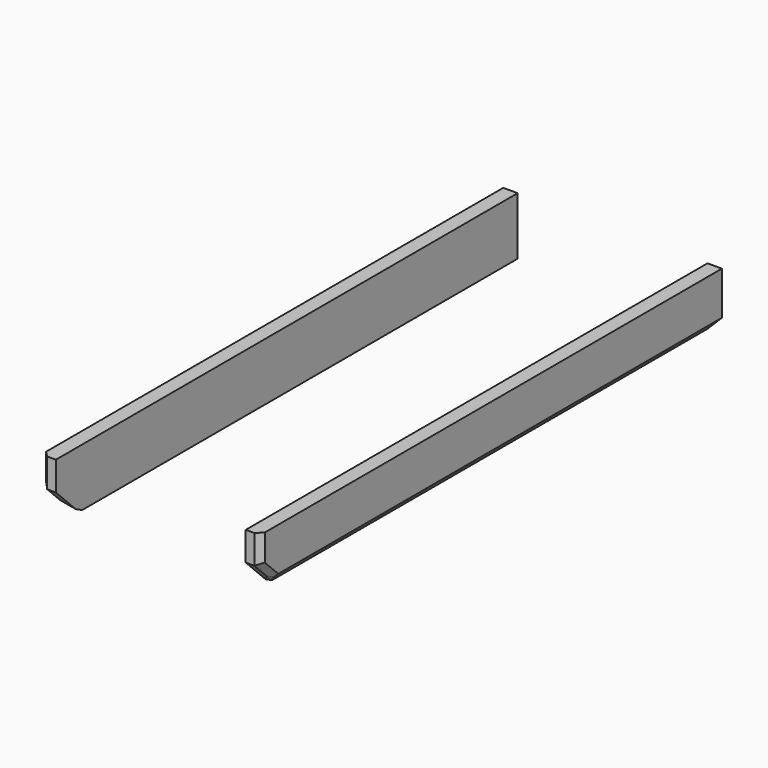
from build123d import *

# Parameters (mm, degrees)
F0_W          = 12.7
F0_H          = 508
F1_DEPTH      = 50.8
F2_SIZE       = 25.4
F4_DEPTH      = 50.8
F5_SIZE       = 25.4
F6_SIZE       = 12.69999
F6_2_SIZE     = 12.69999
F7_T1_DEPTH   = 51.5282991577
F7_T3_DEPTH   = 44.088825542
F7_T5_DEPTH   = 11.4662899398
F7_T7_DEPTH   = 37.54990514
F7_2_T1_DEPTH = 51.5282991577
F7_2_T3_DEPTH = 44.088825542
F7_2_T5_DEPTH = 37.54990514
F7_2_T7_DEPTH = 11.4662899398


# Not quite as in the source:
# - a fillet or chamfer that OpenCascade refuses, or shapes differently, is made with other operations: its cross-section is extruded or revolved along the edge and cut away or added
# - a fillet or chamfer is up to 0.001 mm smaller than in the source, because OpenCascade refuses the exact size
# - a feature of the source that left no trace in its solid (it failed there, or was rolled back) is left out


with BuildPart() as f1:
    # F0 (on Top) → F1 (new body)
    with BuildSketch(Plane.XY):
        Rectangle(F0_W, F0_H)
    extrude(amount=F1_DEPTH)

    # F2
    f2_edges = [f1.edges().sort_by_distance(p)[0] for p in [
        (0, -254, 0),
    ]]
    chamfer(f2_edges, length=F2_SIZE)

    # F6#2 (size 12.7 in the source; OpenCascade refuses exactly that, so slightly less here)
    f6_2_edges = [f1.edges().sort_by_distance(p)[0] for p in [
        (-6.35, 12.7, 0),
    ]]
    chamfer(f6_2_edges, length=F6_2_SIZE)

    # F7: chamfer of 5.08 on 4 edges, made by hand

    # F7_s2 → F7_t1 (cut)
    with BuildSketch(Plane.XY.offset(12.3358504211)):
        Polygon((-6.35, -248.92), (-1.27, -254), (-6.35, -254), align=None)
    extrude(amount=F7_T1_DEPTH, mode=Mode.SUBTRACT)

    # F7_s4 → F7_t3 (cut)
    with BuildSketch(Plane(origin=(0, -148.9377487577, 148.9377487577), x_dir=(1, 0, 0), z_dir=(0, 0.7071067812, -0.7071067812))):
        Polygon((-6.35, 156.5646101792), (-1.27, 161.6446101792), (-6.35, 161.6446101792), align=None)
    extrude(amount=F7_T3_DEPTH, mode=Mode.SUBTRACT)

    # F7_s6 → F7_t5 (cut)
    with BuildSketch(Plane.YZ.offset(0.6168500301)):
        Polygon((-230.0878975516, 1.4878975516), (-226.4957951031, 0), (-228.6, 0), align=None)
    extrude(amount=F7_T5_DEPTH, mode=Mode.SUBTRACT)

    # F7_s8 → F7_t7 (cut)
    with BuildSketch(Plane(origin=(-91.273055587, -91.273055587, 91.273055587), x_dir=(-0.7071067812, 0.7071067812, 0), z_dir=(0.5773502692, 0.5773502692, -0.5773502692))):
        Polygon((-168.6747311687, -89.2667169543), (-163.5947311687, -89.2667169543), (-166.1347311687, -90.7331866381), align=None)
    extrude(amount=F7_T7_DEPTH, mode=Mode.SUBTRACT)


with BuildPart() as f4:
    # F0 (on Top) → F4 (new body)
    with BuildSketch(Plane.XY):
        with Locations((179.7861009836, 0)):
            Rectangle(F0_W, F0_H)
    extrude(amount=F4_DEPTH)

    # F5
    f5_edges = [f4.edges().sort_by_distance(p)[0] for p in [
        (179.786101, -254, 0),
    ]]
    chamfer(f5_edges, length=F5_SIZE)

    # F6 (size 12.7 in the source; OpenCascade refuses exactly that, so slightly less here)
    f6_edges = [f4.edges().sort_by_distance(p)[0] for p in [
        (186.136101, 12.7, 0),
    ]]
    chamfer(f6_edges, length=F6_SIZE)

    # F7#2: chamfer of 5.08 on 4 edges, made by hand

    # F7_2_s2 → F7_2_t1 (cut)
    with BuildSketch(Plane.XY.offset(12.3358504211)):
        Polygon((186.1361009836, -248.92), (181.0561009836, -254), (186.1361009836, -254), align=None)
    extrude(amount=F7_2_T1_DEPTH, mode=Mode.SUBTRACT)

    # F7_2_s4 → F7_2_t3 (cut)
    with BuildSketch(Plane(origin=(0, -148.9377487577, 148.9377487577), x_dir=(1, 0, 0), z_dir=(0, 0.7071067812, -0.7071067812))):
        Polygon((186.1361009836, 156.5646101792), (181.0561009836, 161.6446101792), (186.1361009836, 161.6446101792), align=None)
    extrude(amount=F7_2_T3_DEPTH, mode=Mode.SUBTRACT)

    # F7_2_s6 → F7_2_t5 (cut)
    with BuildSketch(Plane(origin=(151.2017559148, -151.2017559148, 151.2017559148), x_dir=(-0.7071067812, -0.7071067812, 0), z_dir=(-0.5773502692, 0.5773502692, -0.5773502692))):
        Polygon((36.4667600001, -162.6640853301), (41.5467600001, -162.6640853301), (39.0067600001, -164.1305550138), align=None)
    extrude(amount=F7_2_T5_DEPTH, mode=Mode.SUBTRACT)

    # F7_2_s8 → F7_2_t7 (cut)
    with BuildSketch(Plane.YZ.offset(167.7029610137)):
        Polygon((-226.4957951031, 0), (-230.0878975516, 1.4878975516), (-228.6, 0), align=None)
    extrude(amount=F7_2_T7_DEPTH, mode=Mode.SUBTRACT)


solid = Compound([f1.part, f4.part])
